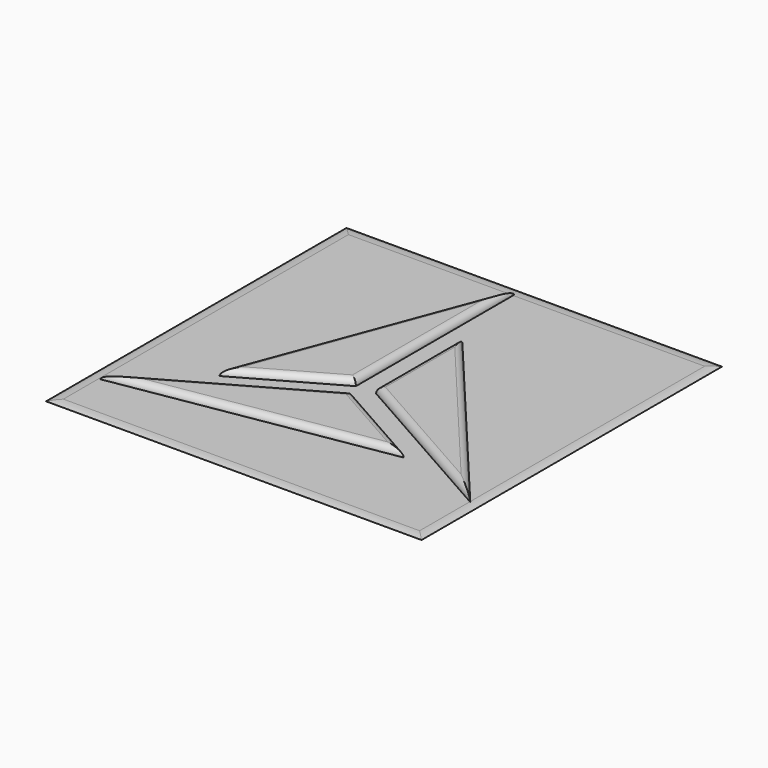
from build123d import *

# Parameters (mm, degrees)
F1_DEPTH    = 1.3
F2_R        = 1.1
F2_2_R      = 1.1
F2_3_R      = 1.1
F4_DEPTH    = 0.2
F5_W        = 65
F5_H        = 65
F6_DEPTH    = 0.2
F7_T1_DEPTH = 73.3066238629
F7_T3_DEPTH = 73.3066238629


# Not quite as in the source:
# - a fillet or chamfer that OpenCascade refuses, or shapes differently, is made with other operations: its cross-section is extruded or revolved along the edge and cut away or added


with BuildPart() as f1:
    # F0 (on Top) → F1 (new body)
    with BuildSketch(Plane.XY):
        Polygon((-24.0248936415, 55.3452231001), (-40.2686429682, 11.9352340698), (-24.0248936415, 21.12738868), align=None)
    extrude(amount=F1_DEPTH)

    # F2
    f2_edges = [f1.edges().sort_by_distance(p)[0] for p in [
        (-32.146768, 33.640229, 1.3),
        (-32.146768, 16.531311, 1.3),
        (-24.024894, 38.236306, 1.3),
    ]]
    fillet(f2_edges, radius=F2_R)


with BuildPart() as f1b:
    # F0 (on Top) → F1, piece 2 (new body)
    with BuildSketch(Plane.XY):
        Polygon((9.2553134576, 4.275105228), (-20.5248936415, 39.791662), (-20.5248936415, 21.12738868), align=None)
    extrude(amount=F1_DEPTH)

    # F2#2
    f2_2_edges = [f1b.edges().sort_by_distance(p)[0] for p in [
        (-5.63479, 22.033384, 1.3),
        (-20.524894, 30.459525, 1.3),
        (-5.63479, 12.701247, 1.3),
    ]]
    fillet(f2_2_edges, radius=F2_2_R)


with BuildPart() as f1c:
    # F0 (on Top) → F1, piece 3 (new body)
    with BuildSketch(Plane.XY):
        Polygon((-52.2528748298, 1.1320981874), (-5.9204182833, 8.8481357249), (-22.2748936415, 18.0962997667), align=None)
    extrude(amount=F1_DEPTH)

    # F2#3
    f2_3_edges = [f1c.edges().sort_by_distance(p)[0] for p in [
        (-29.086647, 4.990117, 1.3),
        (-14.097656, 13.472218, 1.3),
        (-37.263884, 9.614199, 1.3),
    ]]
    fillet(f2_3_edges, radius=F2_3_R)


with BuildPart() as f4:
    # F3 (on face) → F4 (new body)
    with BuildSketch(Plane(origin=(0, 0, 0), x_dir=(1, 0, 0), z_dir=(0, 0, -1))):
        Polygon((-20.5248936415, -39.791662), (9.2553134576, -4.275105228), (-0.4357972381, -9.759195512), (-52.2528104484, -1.1320952326), (-42.1848930418, -6.8243145943), (-24.0248637821, -55.3452596068), (-24.0248637821, -43.9658065178), align=None)
    extrude(amount=-F4_DEPTH)


with BuildPart() as f6:
    # F5 (on Top) → F6 (new body)
    with BuildSketch(Plane.XY):
        with Locations((-21.6999987885, 24.2999990284)):
            Rectangle(F5_W, F5_H)
    extrude(amount=F6_DEPTH)

    # F7: fillet of radius 7 on 4 edges, made by hand

    # F7_s2 → F7_t1 (cut)
    with BuildSketch(Plane.YZ.offset(-58.35331072)):
        with BuildLine():
            ThreePointArc((-8.2000009716, 0), (-7.3753362255, 0.1498201416), (-6.538676199, 0.2))
            Line((-6.538676199, 0.2), (-8.2000009716, 0.2))
            Line((-8.2000009716, 0.2), (-8.2000009716, 0))
        make_face()
        with BuildLine():
            ThreePointArc((56.7999990284, 0), (55.9753342824, 0.1498201416), (55.1386742559, 0.2))
            Line((55.1386742559, 0.2), (56.7999990284, 0.2))
            Line((56.7999990284, 0.2), (56.7999990284, 0))
        make_face()
    extrude(amount=F7_T1_DEPTH, mode=Mode.SUBTRACT)

    # F7_s4 → F7_t3 (cut)
    with BuildSketch(Plane.XZ.offset(-60.9533109599)):
        with BuildLine():
            ThreePointArc((10.8000012115, 0), (9.9753364654, 0.1498201416), (9.1386764389, 0.2))
            Line((9.1386764389, 0.2), (10.8000012115, 0.2))
            Line((10.8000012115, 0.2), (10.8000012115, 0))
        make_face()
        with BuildLine():
            ThreePointArc((-52.538674016, 0.2), (-53.3753340425, 0.1498201416), (-54.1999987885, 0))
            Line((-54.1999987885, 0), (-54.1999987885, 0.2))
            Line((-54.1999987885, 0.2), (-52.538674016, 0.2))
        make_face()
    extrude(amount=F7_T3_DEPTH, mode=Mode.SUBTRACT)


solid = Compound([f1.part, f1b.part, f1c.part, f4.part, f6.part])
